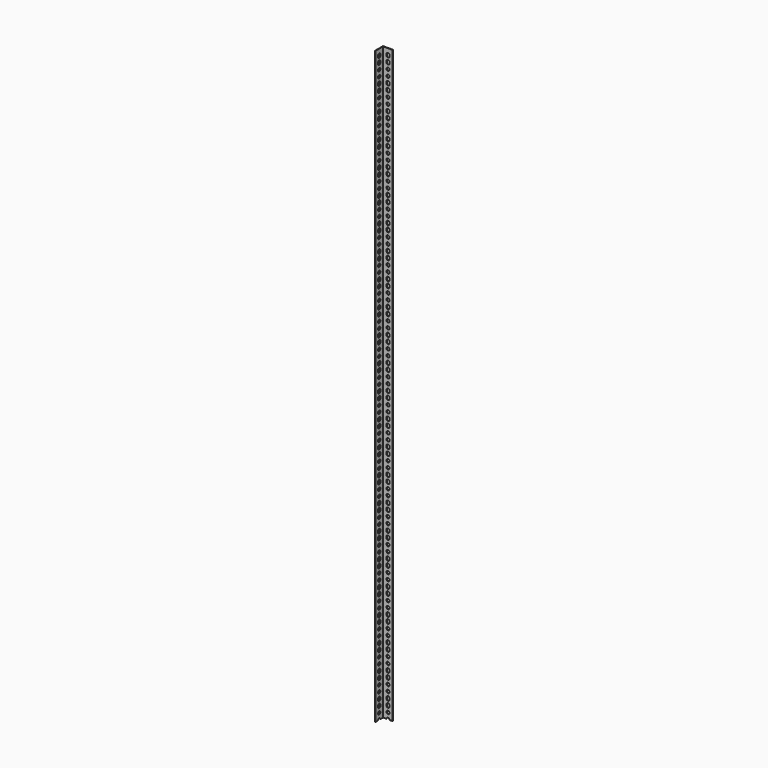
from build123d import *

# Parameters (mm, degrees)
F2_DEPTH = 1828.8
F3_R     = 4.7625
F5_DEPTH = 1.3726
F4_R     = 4.7625
F6_DEPTH = 1.3726


# Not quite as in the source:
# - a variable given as a bare number and used for a length is read in inches; the dataset says mm whatever the document's units were


with BuildPart() as f2:
    # F1 (on Top) → F2 (new body)
    with BuildSketch(Plane.XY):
        Polygon((-1.3716, 1.3716), (-1.3716, -28.7528), (0, -28.7528), (0, 0), (28.7528, 0), (28.7528, 1.3716), align=None)
    extrude(amount=F2_DEPTH)

    # F3 (on face) → F5 (cut, through all)
    with BuildSketch(Plane.XZ):
        with Locations((15.1384, 19.05)):
            Circle(F3_R)
        with Locations((15.1384, 0)):
            Circle(F3_R)
        with BuildLine():
            Line((19.9009, 36.5125), (19.9009, 39.6875))
            ThreePointArc((19.9009, 39.6875), (15.1384, 44.45), (10.3759, 39.6875))
            Line((10.3759, 39.6875), (10.3759, 36.5125))
            ThreePointArc((10.3759, 36.5125), (15.1384, 31.75), (19.9009, 36.5125))
        make_face()
        with BuildLine():
            Line((19.9009, 55.5625), (19.9009, 58.7375))
            ThreePointArc((19.9009, 58.7375), (15.1384, 63.5), (10.3759, 58.7375))
            Line((10.3759, 58.7375), (10.3759, 55.5625))
            ThreePointArc((10.3759, 55.5625), (15.1384, 50.8), (19.9009, 55.5625))
        make_face()
        with BuildLine():
            Line((19.9009, 131.7625), (19.9009, 134.9375))
            ThreePointArc((19.9009, 134.9375), (15.1384, 139.7), (10.3759, 134.9375))
            Line((10.3759, 134.9375), (10.3759, 131.7625))
            ThreePointArc((10.3759, 131.7625), (15.1384, 127), (19.9009, 131.7625))
        make_face()
        with Locations((15.1384, 95.25)):
            Circle(F3_R)
        with Locations((15.1384, 76.2)):
            Circle(F3_R)
        with BuildLine():
            Line((19.9009, 112.7125), (19.9009, 115.8875))
            ThreePointArc((19.9009, 115.8875), (15.1384, 120.65), (10.3759, 115.8875))
            Line((10.3759, 115.8875), (10.3759, 112.7125))
            ThreePointArc((10.3759, 112.7125), (15.1384, 107.95), (19.9009, 112.7125))
        make_face()
        with BuildLine():
            Line((19.9009, 207.9625), (19.9009, 211.1375))
            ThreePointArc((19.9009, 211.1375), (15.1384, 215.9), (10.3759, 211.1375))
            Line((10.3759, 211.1375), (10.3759, 207.9625))
            ThreePointArc((10.3759, 207.9625), (15.1384, 203.2), (19.9009, 207.9625))
        make_face()
        with Locations((15.1384, 171.45)):
            Circle(F3_R)
        with Locations((15.1384, 152.4)):
            Circle(F3_R)
        with BuildLine():
            Line((19.9009, 188.9125), (19.9009, 192.0875))
            ThreePointArc((19.9009, 192.0875), (15.1384, 196.85), (10.3759, 192.0875))
            Line((10.3759, 192.0875), (10.3759, 188.9125))
            ThreePointArc((10.3759, 188.9125), (15.1384, 184.15), (19.9009, 188.9125))
        make_face()
        with BuildLine():
            Line((19.9009, 284.1625), (19.9009, 287.3375))
            ThreePointArc((19.9009, 287.3375), (15.1384, 292.1), (10.3759, 287.3375))
            Line((10.3759, 287.3375), (10.3759, 284.1625))
            ThreePointArc((10.3759, 284.1625), (15.1384, 279.4), (19.9009, 284.1625))
        make_face()
        with Locations((15.1384, 247.65)):
            Circle(F3_R)
        with Locations((15.1384, 228.6)):
            Circle(F3_R)
        with BuildLine():
            Line((19.9009, 265.1125), (19.9009, 268.2875))
            ThreePointArc((19.9009, 268.2875), (15.1384, 273.05), (10.3759, 268.2875))
            Line((10.3759, 268.2875), (10.3759, 265.1125))
            ThreePointArc((10.3759, 265.1125), (15.1384, 260.35), (19.9009, 265.1125))
        make_face()
        with BuildLine():
            Line((19.9009, 360.3625), (19.9009, 363.5375))
            ThreePointArc((19.9009, 363.5375), (15.1384, 368.3), (10.3759, 363.5375))
            Line((10.3759, 363.5375), (10.3759, 360.3625))
            ThreePointArc((10.3759, 360.3625), (15.1384, 355.6), (19.9009, 360.3625))
        make_face()
        with Locations((15.1384, 323.85)):
            Circle(F3_R)
        with Locations((15.1384, 304.8)):
            Circle(F3_R)
        with BuildLine():
            Line((19.9009, 341.3125), (19.9009, 344.4875))
            ThreePointArc((19.9009, 344.4875), (15.1384, 349.25), (10.3759, 344.4875))
            Line((10.3759, 344.4875), (10.3759, 341.3125))
            ThreePointArc((10.3759, 341.3125), (15.1384, 336.55), (19.9009, 341.3125))
        make_face()
        with BuildLine():
            Line((19.9009, 436.5625), (19.9009, 439.7375))
            ThreePointArc((19.9009, 439.7375), (15.1384, 444.5), (10.3759, 439.7375))
            Line((10.3759, 439.7375), (10.3759, 436.5625))
            ThreePointArc((10.3759, 436.5625), (15.1384, 431.8), (19.9009, 436.5625))
        make_face()
        with Locations((15.1384, 400.05)):
            Circle(F3_R)
        with Locations((15.1384, 381)):
            Circle(F3_R)
        with BuildLine():
            Line((19.9009, 417.5125), (19.9009, 420.6875))
            ThreePointArc((19.9009, 420.6875), (15.1384, 425.45), (10.3759, 420.6875))
            Line((10.3759, 420.6875), (10.3759, 417.5125))
            ThreePointArc((10.3759, 417.5125), (15.1384, 412.75), (19.9009, 417.5125))
        make_face()
        with BuildLine():
            Line((19.9009, 512.7625), (19.9009, 515.9375))
            ThreePointArc((19.9009, 515.9375), (15.1384, 520.7), (10.3759, 515.9375))
            Line((10.3759, 515.9375), (10.3759, 512.7625))
            ThreePointArc((10.3759, 512.7625), (15.1384, 508), (19.9009, 512.7625))
        make_face()
        with Locations((15.1384, 476.25)):
            Circle(F3_R)
        with Locations((15.1384, 457.2)):
            Circle(F3_R)
        with BuildLine():
            Line((19.9009, 493.7125), (19.9009, 496.8875))
            ThreePointArc((19.9009, 496.8875), (15.1384, 501.65), (10.3759, 496.8875))
            Line((10.3759, 496.8875), (10.3759, 493.7125))
            ThreePointArc((10.3759, 493.7125), (15.1384, 488.95), (19.9009, 493.7125))
        make_face()
        with BuildLine():
            Line((19.9009, 588.9625), (19.9009, 592.1375))
            ThreePointArc((19.9009, 592.1375), (15.1384, 596.9), (10.3759, 592.1375))
            Line((10.3759, 592.1375), (10.3759, 588.9625))
            ThreePointArc((10.3759, 588.9625), (15.1384, 584.2), (19.9009, 588.9625))
        make_face()
        with Locations((15.1384, 552.45)):
            Circle(F3_R)
        with Locations((15.1384, 533.4)):
            Circle(F3_R)
        with BuildLine():
            Line((19.9009, 569.9125), (19.9009, 573.0875))
            ThreePointArc((19.9009, 573.0875), (15.1384, 577.85), (10.3759, 573.0875))
            Line((10.3759, 573.0875), (10.3759, 569.9125))
            ThreePointArc((10.3759, 569.9125), (15.1384, 565.15), (19.9009, 569.9125))
        make_face()
        with BuildLine():
            Line((19.9009, 665.1625), (19.9009, 668.3375))
            ThreePointArc((19.9009, 668.3375), (15.1384, 673.1), (10.3759, 668.3375))
            Line((10.3759, 668.3375), (10.3759, 665.1625))
            ThreePointArc((10.3759, 665.1625), (15.1384, 660.4), (19.9009, 665.1625))
        make_face()
        with Locations((15.1384, 628.65)):
            Circle(F3_R)
        with Locations((15.1384, 609.6)):
            Circle(F3_R)
        with BuildLine():
            Line((19.9009, 646.1125), (19.9009, 649.2875))
            ThreePointArc((19.9009, 649.2875), (15.1384, 654.05), (10.3759, 649.2875))
            Line((10.3759, 649.2875), (10.3759, 646.1125))
            ThreePointArc((10.3759, 646.1125), (15.1384, 641.35), (19.9009, 646.1125))
        make_face()
        with BuildLine():
            Line((19.9009, 741.3625), (19.9009, 744.5375))
            ThreePointArc((19.9009, 744.5375), (15.1384, 749.3), (10.3759, 744.5375))
            Line((10.3759, 744.5375), (10.3759, 741.3625))
            ThreePointArc((10.3759, 741.3625), (15.1384, 736.6), (19.9009, 741.3625))
        make_face()
        with Locations((15.1384, 704.85)):
            Circle(F3_R)
        with Locations((15.1384, 685.8)):
            Circle(F3_R)
        with BuildLine():
            Line((19.9009, 722.3125), (19.9009, 725.4875))
            ThreePointArc((19.9009, 725.4875), (15.1384, 730.25), (10.3759, 725.4875))
            Line((10.3759, 725.4875), (10.3759, 722.3125))
            ThreePointArc((10.3759, 722.3125), (15.1384, 717.55), (19.9009, 722.3125))
        make_face()
        with BuildLine():
            Line((19.9009, 817.5625), (19.9009, 820.7375))
            ThreePointArc((19.9009, 820.7375), (15.1384, 825.5), (10.3759, 820.7375))
            Line((10.3759, 820.7375), (10.3759, 817.5625))
            ThreePointArc((10.3759, 817.5625), (15.1384, 812.8), (19.9009, 817.5625))
        make_face()
        with Locations((15.1384, 781.05)):
            Circle(F3_R)
        with Locations((15.1384, 762)):
            Circle(F3_R)
        with BuildLine():
            Line((19.9009, 798.5125), (19.9009, 801.6875))
            ThreePointArc((19.9009, 801.6875), (15.1384, 806.45), (10.3759, 801.6875))
            Line((10.3759, 801.6875), (10.3759, 798.5125))
            ThreePointArc((10.3759, 798.5125), (15.1384, 793.75), (19.9009, 798.5125))
        make_face()
        with BuildLine():
            Line((19.9009, 893.7625), (19.9009, 896.9375))
            ThreePointArc((19.9009, 896.9375), (15.1384, 901.7), (10.3759, 896.9375))
            Line((10.3759, 896.9375), (10.3759, 893.7625))
            ThreePointArc((10.3759, 893.7625), (15.1384, 889), (19.9009, 893.7625))
        make_face()
        with Locations((15.1384, 857.25)):
            Circle(F3_R)
        with Locations((15.1384, 838.2)):
            Circle(F3_R)
        with BuildLine():
            Line((19.9009, 874.7125), (19.9009, 877.8875))
            ThreePointArc((19.9009, 877.8875), (15.1384, 882.65), (10.3759, 877.8875))
            Line((10.3759, 877.8875), (10.3759, 874.7125))
            ThreePointArc((10.3759, 874.7125), (15.1384, 869.95), (19.9009, 874.7125))
        make_face()
        with BuildLine():
            Line((19.9009, 969.9625), (19.9009, 973.1375))
            ThreePointArc((19.9009, 973.1375), (15.1384, 977.9), (10.3759, 973.1375))
            Line((10.3759, 973.1375), (10.3759, 969.9625))
            ThreePointArc((10.3759, 969.9625), (15.1384, 965.2), (19.9009, 969.9625))
        make_face()
        with Locations((15.1384, 933.45)):
            Circle(F3_R)
        with Locations((15.1384, 914.4)):
            Circle(F3_R)
        with BuildLine():
            Line((19.9009, 950.9125), (19.9009, 954.0875))
            ThreePointArc((19.9009, 954.0875), (15.1384, 958.85), (10.3759, 954.0875))
            Line((10.3759, 954.0875), (10.3759, 950.9125))
            ThreePointArc((10.3759, 950.9125), (15.1384, 946.15), (19.9009, 950.9125))
        make_face()
        with BuildLine():
            Line((19.9009, 1046.1625), (19.9009, 1049.3375))
            ThreePointArc((19.9009, 1049.3375), (15.1384, 1054.1), (10.3759, 1049.3375))
            Line((10.3759, 1049.3375), (10.3759, 1046.1625))
            ThreePointArc((10.3759, 1046.1625), (15.1384, 1041.4), (19.9009, 1046.1625))
        make_face()
        with Locations((15.1384, 1009.65)):
            Circle(F3_R)
        with Locations((15.1384, 990.6)):
            Circle(F3_R)
        with BuildLine():
            Line((19.9009, 1027.1125), (19.9009, 1030.2875))
            ThreePointArc((19.9009, 1030.2875), (15.1384, 1035.05), (10.3759, 1030.2875))
            Line((10.3759, 1030.2875), (10.3759, 1027.1125))
            ThreePointArc((10.3759, 1027.1125), (15.1384, 1022.35), (19.9009, 1027.1125))
        make_face()
        with BuildLine():
            Line((19.9009, 1122.3625), (19.9009, 1125.5375))
            ThreePointArc((19.9009, 1125.5375), (15.1384, 1130.3), (10.3759, 1125.5375))
            Line((10.3759, 1125.5375), (10.3759, 1122.3625))
            ThreePointArc((10.3759, 1122.3625), (15.1384, 1117.6), (19.9009, 1122.3625))
        make_face()
        with Locations((15.1384, 1085.85)):
            Circle(F3_R)
        with Locations((15.1384, 1066.8)):
            Circle(F3_R)
        with BuildLine():
            Line((19.9009, 1103.3125), (19.9009, 1106.4875))
            ThreePointArc((19.9009, 1106.4875), (15.1384, 1111.25), (10.3759, 1106.4875))
            Line((10.3759, 1106.4875), (10.3759, 1103.3125))
            ThreePointArc((10.3759, 1103.3125), (15.1384, 1098.55), (19.9009, 1103.3125))
        make_face()
        with BuildLine():
            Line((19.9009, 1198.5625), (19.9009, 1201.7375))
            ThreePointArc((19.9009, 1201.7375), (15.1384, 1206.5), (10.3759, 1201.7375))
            Line((10.3759, 1201.7375), (10.3759, 1198.5625))
            ThreePointArc((10.3759, 1198.5625), (15.1384, 1193.8), (19.9009, 1198.5625))
        make_face()
        with Locations((15.1384, 1162.05)):
            Circle(F3_R)
        with Locations((15.1384, 1143)):
            Circle(F3_R)
        with BuildLine():
            Line((19.9009, 1179.5125), (19.9009, 1182.6875))
            ThreePointArc((19.9009, 1182.6875), (15.1384, 1187.45), (10.3759, 1182.6875))
            Line((10.3759, 1182.6875), (10.3759, 1179.5125))
            ThreePointArc((10.3759, 1179.5125), (15.1384, 1174.75), (19.9009, 1179.5125))
        make_face()
        with BuildLine():
            Line((19.9009, 1274.7625), (19.9009, 1277.9375))
            ThreePointArc((19.9009, 1277.9375), (15.1384, 1282.7), (10.3759, 1277.9375))
            Line((10.3759, 1277.9375), (10.3759, 1274.7625))
            ThreePointArc((10.3759, 1274.7625), (15.1384, 1270), (19.9009, 1274.7625))
        make_face()
        with Locations((15.1384, 1238.25)):
            Circle(F3_R)
        with Locations((15.1384, 1219.2)):
            Circle(F3_R)
        with BuildLine():
            Line((19.9009, 1255.7125), (19.9009, 1258.8875))
            ThreePointArc((19.9009, 1258.8875), (15.1384, 1263.65), (10.3759, 1258.8875))
            Line((10.3759, 1258.8875), (10.3759, 1255.7125))
            ThreePointArc((10.3759, 1255.7125), (15.1384, 1250.95), (19.9009, 1255.7125))
        make_face()
        with BuildLine():
            Line((19.9009, 1350.9625), (19.9009, 1354.1375))
            ThreePointArc((19.9009, 1354.1375), (15.1384, 1358.9), (10.3759, 1354.1375))
            Line((10.3759, 1354.1375), (10.3759, 1350.9625))
            ThreePointArc((10.3759, 1350.9625), (15.1384, 1346.2), (19.9009, 1350.9625))
        make_face()
        with Locations((15.1384, 1314.45)):
            Circle(F3_R)
        with Locations((15.1384, 1295.4)):
            Circle(F3_R)
        with BuildLine():
            Line((19.9009, 1331.9125), (19.9009, 1335.0875))
            ThreePointArc((19.9009, 1335.0875), (15.1384, 1339.85), (10.3759, 1335.0875))
            Line((10.3759, 1335.0875), (10.3759, 1331.9125))
            ThreePointArc((10.3759, 1331.9125), (15.1384, 1327.15), (19.9009, 1331.9125))
        make_face()
        with BuildLine():
            Line((19.9009, 1427.1625), (19.9009, 1430.3375))
            ThreePointArc((19.9009, 1430.3375), (15.1384, 1435.1), (10.3759, 1430.3375))
            Line((10.3759, 1430.3375), (10.3759, 1427.1625))
            ThreePointArc((10.3759, 1427.1625), (15.1384, 1422.4), (19.9009, 1427.1625))
        make_face()
        with Locations((15.1384, 1390.65)):
            Circle(F3_R)
        with Locations((15.1384, 1371.6)):
            Circle(F3_R)
        with BuildLine():
            Line((19.9009, 1408.1125), (19.9009, 1411.2875))
            ThreePointArc((19.9009, 1411.2875), (15.1384, 1416.05), (10.3759, 1411.2875))
            Line((10.3759, 1411.2875), (10.3759, 1408.1125))
            ThreePointArc((10.3759, 1408.1125), (15.1384, 1403.35), (19.9009, 1408.1125))
        make_face()
        with BuildLine():
            Line((19.9009, 1503.3625), (19.9009, 1506.5375))
            ThreePointArc((19.9009, 1506.5375), (15.1384, 1511.3), (10.3759, 1506.5375))
            Line((10.3759, 1506.5375), (10.3759, 1503.3625))
            ThreePointArc((10.3759, 1503.3625), (15.1384, 1498.6), (19.9009, 1503.3625))
        make_face()
        with Locations((15.1384, 1466.85)):
            Circle(F3_R)
        with Locations((15.1384, 1447.8)):
            Circle(F3_R)
        with BuildLine():
            Line((19.9009, 1484.3125), (19.9009, 1487.4875))
            ThreePointArc((19.9009, 1487.4875), (15.1384, 1492.25), (10.3759, 1487.4875))
            Line((10.3759, 1487.4875), (10.3759, 1484.3125))
            ThreePointArc((10.3759, 1484.3125), (15.1384, 1479.55), (19.9009, 1484.3125))
        make_face()
        with BuildLine():
            Line((19.9009, 1579.5625), (19.9009, 1582.7375))
            ThreePointArc((19.9009, 1582.7375), (15.1384, 1587.5), (10.3759, 1582.7375))
            Line((10.3759, 1582.7375), (10.3759, 1579.5625))
            ThreePointArc((10.3759, 1579.5625), (15.1384, 1574.8), (19.9009, 1579.5625))
        make_face()
        with Locations((15.1384, 1543.05)):
            Circle(F3_R)
        with Locations((15.1384, 1524)):
            Circle(F3_R)
        with BuildLine():
            Line((19.9009, 1560.5125), (19.9009, 1563.6875))
            ThreePointArc((19.9009, 1563.6875), (15.1384, 1568.45), (10.3759, 1563.6875))
            Line((10.3759, 1563.6875), (10.3759, 1560.5125))
            ThreePointArc((10.3759, 1560.5125), (15.1384, 1555.75), (19.9009, 1560.5125))
        make_face()
        with BuildLine():
            Line((19.9009, 1655.7625), (19.9009, 1658.9375))
            ThreePointArc((19.9009, 1658.9375), (15.1384, 1663.7), (10.3759, 1658.9375))
            Line((10.3759, 1658.9375), (10.3759, 1655.7625))
            ThreePointArc((10.3759, 1655.7625), (15.1384, 1651), (19.9009, 1655.7625))
        make_face()
        with Locations((15.1384, 1619.25)):
            Circle(F3_R)
        with Locations((15.1384, 1600.2)):
            Circle(F3_R)
        with BuildLine():
            Line((19.9009, 1636.7125), (19.9009, 1639.8875))
            ThreePointArc((19.9009, 1639.8875), (15.1384, 1644.65), (10.3759, 1639.8875))
            Line((10.3759, 1639.8875), (10.3759, 1636.7125))
            ThreePointArc((10.3759, 1636.7125), (15.1384, 1631.95), (19.9009, 1636.7125))
        make_face()
        with BuildLine():
            Line((19.9009, 1731.9625), (19.9009, 1735.1375))
            ThreePointArc((19.9009, 1735.1375), (15.1384, 1739.9), (10.3759, 1735.1375))
            Line((10.3759, 1735.1375), (10.3759, 1731.9625))
            ThreePointArc((10.3759, 1731.9625), (15.1384, 1727.2), (19.9009, 1731.9625))
        make_face()
        with Locations((15.1384, 1695.45)):
            Circle(F3_R)
        with Locations((15.1384, 1676.4)):
            Circle(F3_R)
        with BuildLine():
            Line((19.9009, 1712.9125), (19.9009, 1716.0875))
            ThreePointArc((19.9009, 1716.0875), (15.1384, 1720.85), (10.3759, 1716.0875))
            Line((10.3759, 1716.0875), (10.3759, 1712.9125))
            ThreePointArc((10.3759, 1712.9125), (15.1384, 1708.15), (19.9009, 1712.9125))
        make_face()
        with BuildLine():
            Line((19.9009, 1808.1625), (19.9009, 1811.3375))
            ThreePointArc((19.9009, 1811.3375), (15.1384, 1816.1), (10.3759, 1811.3375))
            Line((10.3759, 1811.3375), (10.3759, 1808.1625))
            ThreePointArc((10.3759, 1808.1625), (15.1384, 1803.4), (19.9009, 1808.1625))
        make_face()
        with Locations((15.1384, 1771.65)):
            Circle(F3_R)
        with Locations((15.1384, 1752.6)):
            Circle(F3_R)
        with BuildLine():
            Line((19.9009, 1789.1125), (19.9009, 1792.2875))
            ThreePointArc((19.9009, 1792.2875), (15.1384, 1797.05), (10.3759, 1792.2875))
            Line((10.3759, 1792.2875), (10.3759, 1789.1125))
            ThreePointArc((10.3759, 1789.1125), (15.1384, 1784.35), (19.9009, 1789.1125))
        make_face()
    extrude(amount=-F5_DEPTH, mode=Mode.SUBTRACT)

    # F4 (on face) → F6 (cut, through all)
    with BuildSketch(Plane.YZ):
        with Locations((-15.1384, 19.05)):
            Circle(F4_R)
        with Locations((-15.1384, 0)):
            Circle(F4_R)
        with BuildLine():
            Line((-10.3759, 36.5125), (-10.3759, 39.6875))
            ThreePointArc((-10.3759, 39.6875), (-15.1384, 44.45), (-19.9009, 39.6875))
            Line((-19.9009, 39.6875), (-19.9009, 36.5125))
            ThreePointArc((-19.9009, 36.5125), (-15.1384, 31.75), (-10.3759, 36.5125))
        make_face()
        with BuildLine():
            Line((-10.3759, 55.5625), (-10.3759, 58.7375))
            ThreePointArc((-10.3759, 58.7375), (-15.1384, 63.5), (-19.9009, 58.7375))
            Line((-19.9009, 58.7375), (-19.9009, 55.5625))
            ThreePointArc((-19.9009, 55.5625), (-15.1384, 50.8), (-10.3759, 55.5625))
        make_face()
        with BuildLine():
            Line((-10.3759, 131.7625), (-10.3759, 134.9375))
            ThreePointArc((-10.3759, 134.9375), (-15.1384, 139.7), (-19.9009, 134.9375))
            Line((-19.9009, 134.9375), (-19.9009, 131.7625))
            ThreePointArc((-19.9009, 131.7625), (-15.1384, 127), (-10.3759, 131.7625))
        make_face()
        with Locations((-15.1384, 95.25)):
            Circle(F4_R)
        with Locations((-15.1384, 76.2)):
            Circle(F4_R)
        with BuildLine():
            Line((-10.3759, 112.7125), (-10.3759, 115.8875))
            ThreePointArc((-10.3759, 115.8875), (-15.1384, 120.65), (-19.9009, 115.8875))
            Line((-19.9009, 115.8875), (-19.9009, 112.7125))
            ThreePointArc((-19.9009, 112.7125), (-15.1384, 107.95), (-10.3759, 112.7125))
        make_face()
        with BuildLine():
            Line((-10.3759, 207.9625), (-10.3759, 211.1375))
            ThreePointArc((-10.3759, 211.1375), (-15.1384, 215.9), (-19.9009, 211.1375))
            Line((-19.9009, 211.1375), (-19.9009, 207.9625))
            ThreePointArc((-19.9009, 207.9625), (-15.1384, 203.2), (-10.3759, 207.9625))
        make_face()
        with Locations((-15.1384, 171.45)):
            Circle(F4_R)
        with Locations((-15.1384, 152.4)):
            Circle(F4_R)
        with BuildLine():
            Line((-10.3759, 188.9125), (-10.3759, 192.0875))
            ThreePointArc((-10.3759, 192.0875), (-15.1384, 196.85), (-19.9009, 192.0875))
            Line((-19.9009, 192.0875), (-19.9009, 188.9125))
            ThreePointArc((-19.9009, 188.9125), (-15.1384, 184.15), (-10.3759, 188.9125))
        make_face()
        with BuildLine():
            Line((-10.3759, 284.1625), (-10.3759, 287.3375))
            ThreePointArc((-10.3759, 287.3375), (-15.1384, 292.1), (-19.9009, 287.3375))
            Line((-19.9009, 287.3375), (-19.9009, 284.1625))
            ThreePointArc((-19.9009, 284.1625), (-15.1384, 279.4), (-10.3759, 284.1625))
        make_face()
        with Locations((-15.1384, 247.65)):
            Circle(F4_R)
        with Locations((-15.1384, 228.6)):
            Circle(F4_R)
        with BuildLine():
            Line((-10.3759, 265.1125), (-10.3759, 268.2875))
            ThreePointArc((-10.3759, 268.2875), (-15.1384, 273.05), (-19.9009, 268.2875))
            Line((-19.9009, 268.2875), (-19.9009, 265.1125))
            ThreePointArc((-19.9009, 265.1125), (-15.1384, 260.35), (-10.3759, 265.1125))
        make_face()
        with BuildLine():
            Line((-10.3759, 360.3625), (-10.3759, 363.5375))
            ThreePointArc((-10.3759, 363.5375), (-15.1384, 368.3), (-19.9009, 363.5375))
            Line((-19.9009, 363.5375), (-19.9009, 360.3625))
            ThreePointArc((-19.9009, 360.3625), (-15.1384, 355.6), (-10.3759, 360.3625))
        make_face()
        with Locations((-15.1384, 323.85)):
            Circle(F4_R)
        with Locations((-15.1384, 304.8)):
            Circle(F4_R)
        with BuildLine():
            Line((-10.3759, 341.3125), (-10.3759, 344.4875))
            ThreePointArc((-10.3759, 344.4875), (-15.1384, 349.25), (-19.9009, 344.4875))
            Line((-19.9009, 344.4875), (-19.9009, 341.3125))
            ThreePointArc((-19.9009, 341.3125), (-15.1384, 336.55), (-10.3759, 341.3125))
        make_face()
        with BuildLine():
            Line((-10.3759, 436.5625), (-10.3759, 439.7375))
            ThreePointArc((-10.3759, 439.7375), (-15.1384, 444.5), (-19.9009, 439.7375))
            Line((-19.9009, 439.7375), (-19.9009, 436.5625))
            ThreePointArc((-19.9009, 436.5625), (-15.1384, 431.8), (-10.3759, 436.5625))
        make_face()
        with Locations((-15.1384, 400.05)):
            Circle(F4_R)
        with Locations((-15.1384, 381)):
            Circle(F4_R)
        with BuildLine():
            Line((-10.3759, 417.5125), (-10.3759, 420.6875))
            ThreePointArc((-10.3759, 420.6875), (-15.1384, 425.45), (-19.9009, 420.6875))
            Line((-19.9009, 420.6875), (-19.9009, 417.5125))
            ThreePointArc((-19.9009, 417.5125), (-15.1384, 412.75), (-10.3759, 417.5125))
        make_face()
        with BuildLine():
            Line((-10.3759, 512.7625), (-10.3759, 515.9375))
            ThreePointArc((-10.3759, 515.9375), (-15.1384, 520.7), (-19.9009, 515.9375))
            Line((-19.9009, 515.9375), (-19.9009, 512.7625))
            ThreePointArc((-19.9009, 512.7625), (-15.1384, 508), (-10.3759, 512.7625))
        make_face()
        with Locations((-15.1384, 476.25)):
            Circle(F4_R)
        with Locations((-15.1384, 457.2)):
            Circle(F4_R)
        with BuildLine():
            Line((-10.3759, 493.7125), (-10.3759, 496.8875))
            ThreePointArc((-10.3759, 496.8875), (-15.1384, 501.65), (-19.9009, 496.8875))
            Line((-19.9009, 496.8875), (-19.9009, 493.7125))
            ThreePointArc((-19.9009, 493.7125), (-15.1384, 488.95), (-10.3759, 493.7125))
        make_face()
        with BuildLine():
            Line((-10.3759, 588.9625), (-10.3759, 592.1375))
            ThreePointArc((-10.3759, 592.1375), (-15.1384, 596.9), (-19.9009, 592.1375))
            Line((-19.9009, 592.1375), (-19.9009, 588.9625))
            ThreePointArc((-19.9009, 588.9625), (-15.1384, 584.2), (-10.3759, 588.9625))
        make_face()
        with Locations((-15.1384, 552.45)):
            Circle(F4_R)
        with Locations((-15.1384, 533.4)):
            Circle(F4_R)
        with BuildLine():
            Line((-10.3759, 569.9125), (-10.3759, 573.0875))
            ThreePointArc((-10.3759, 573.0875), (-15.1384, 577.85), (-19.9009, 573.0875))
            Line((-19.9009, 573.0875), (-19.9009, 569.9125))
            ThreePointArc((-19.9009, 569.9125), (-15.1384, 565.15), (-10.3759, 569.9125))
        make_face()
        with BuildLine():
            Line((-10.3759, 665.1625), (-10.3759, 668.3375))
            ThreePointArc((-10.3759, 668.3375), (-15.1384, 673.1), (-19.9009, 668.3375))
            Line((-19.9009, 668.3375), (-19.9009, 665.1625))
            ThreePointArc((-19.9009, 665.1625), (-15.1384, 660.4), (-10.3759, 665.1625))
        make_face()
        with Locations((-15.1384, 628.65)):
            Circle(F4_R)
        with Locations((-15.1384, 609.6)):
            Circle(F4_R)
        with BuildLine():
            Line((-10.3759, 646.1125), (-10.3759, 649.2875))
            ThreePointArc((-10.3759, 649.2875), (-15.1384, 654.05), (-19.9009, 649.2875))
            Line((-19.9009, 649.2875), (-19.9009, 646.1125))
            ThreePointArc((-19.9009, 646.1125), (-15.1384, 641.35), (-10.3759, 646.1125))
        make_face()
        with BuildLine():
            Line((-10.3759, 741.3625), (-10.3759, 744.5375))
            ThreePointArc((-10.3759, 744.5375), (-15.1384, 749.3), (-19.9009, 744.5375))
            Line((-19.9009, 744.5375), (-19.9009, 741.3625))
            ThreePointArc((-19.9009, 741.3625), (-15.1384, 736.6), (-10.3759, 741.3625))
        make_face()
        with Locations((-15.1384, 704.85)):
            Circle(F4_R)
        with Locations((-15.1384, 685.8)):
            Circle(F4_R)
        with BuildLine():
            Line((-10.3759, 722.3125), (-10.3759, 725.4875))
            ThreePointArc((-10.3759, 725.4875), (-15.1384, 730.25), (-19.9009, 725.4875))
            Line((-19.9009, 725.4875), (-19.9009, 722.3125))
            ThreePointArc((-19.9009, 722.3125), (-15.1384, 717.55), (-10.3759, 722.3125))
        make_face()
        with BuildLine():
            Line((-10.3759, 817.5625), (-10.3759, 820.7375))
            ThreePointArc((-10.3759, 820.7375), (-15.1384, 825.5), (-19.9009, 820.7375))
            Line((-19.9009, 820.7375), (-19.9009, 817.5625))
            ThreePointArc((-19.9009, 817.5625), (-15.1384, 812.8), (-10.3759, 817.5625))
        make_face()
        with Locations((-15.1384, 781.05)):
            Circle(F4_R)
        with Locations((-15.1384, 762)):
            Circle(F4_R)
        with BuildLine():
            Line((-10.3759, 798.5125), (-10.3759, 801.6875))
            ThreePointArc((-10.3759, 801.6875), (-15.1384, 806.45), (-19.9009, 801.6875))
            Line((-19.9009, 801.6875), (-19.9009, 798.5125))
            ThreePointArc((-19.9009, 798.5125), (-15.1384, 793.75), (-10.3759, 798.5125))
        make_face()
        with BuildLine():
            Line((-10.3759, 893.7625), (-10.3759, 896.9375))
            ThreePointArc((-10.3759, 896.9375), (-15.1384, 901.7), (-19.9009, 896.9375))
            Line((-19.9009, 896.9375), (-19.9009, 893.7625))
            ThreePointArc((-19.9009, 893.7625), (-15.1384, 889), (-10.3759, 893.7625))
        make_face()
        with Locations((-15.1384, 857.25)):
            Circle(F4_R)
        with Locations((-15.1384, 838.2)):
            Circle(F4_R)
        with BuildLine():
            Line((-10.3759, 874.7125), (-10.3759, 877.8875))
            ThreePointArc((-10.3759, 877.8875), (-15.1384, 882.65), (-19.9009, 877.8875))
            Line((-19.9009, 877.8875), (-19.9009, 874.7125))
            ThreePointArc((-19.9009, 874.7125), (-15.1384, 869.95), (-10.3759, 874.7125))
        make_face()
        with BuildLine():
            Line((-10.3759, 969.9625), (-10.3759, 973.1375))
            ThreePointArc((-10.3759, 973.1375), (-15.1384, 977.9), (-19.9009, 973.1375))
            Line((-19.9009, 973.1375), (-19.9009, 969.9625))
            ThreePointArc((-19.9009, 969.9625), (-15.1384, 965.2), (-10.3759, 969.9625))
        make_face()
        with Locations((-15.1384, 933.45)):
            Circle(F4_R)
        with Locations((-15.1384, 914.4)):
            Circle(F4_R)
        with BuildLine():
            Line((-10.3759, 950.9125), (-10.3759, 954.0875))
            ThreePointArc((-10.3759, 954.0875), (-15.1384, 958.85), (-19.9009, 954.0875))
            Line((-19.9009, 954.0875), (-19.9009, 950.9125))
            ThreePointArc((-19.9009, 950.9125), (-15.1384, 946.15), (-10.3759, 950.9125))
        make_face()
        with BuildLine():
            Line((-10.3759, 1046.1625), (-10.3759, 1049.3375))
            ThreePointArc((-10.3759, 1049.3375), (-15.1384, 1054.1), (-19.9009, 1049.3375))
            Line((-19.9009, 1049.3375), (-19.9009, 1046.1625))
            ThreePointArc((-19.9009, 1046.1625), (-15.1384, 1041.4), (-10.3759, 1046.1625))
        make_face()
        with Locations((-15.1384, 1009.65)):
            Circle(F4_R)
        with Locations((-15.1384, 990.6)):
            Circle(F4_R)
        with BuildLine():
            Line((-10.3759, 1027.1125), (-10.3759, 1030.2875))
            ThreePointArc((-10.3759, 1030.2875), (-15.1384, 1035.05), (-19.9009, 1030.2875))
            Line((-19.9009, 1030.2875), (-19.9009, 1027.1125))
            ThreePointArc((-19.9009, 1027.1125), (-15.1384, 1022.35), (-10.3759, 1027.1125))
        make_face()
        with BuildLine():
            Line((-10.3759, 1122.3625), (-10.3759, 1125.5375))
            ThreePointArc((-10.3759, 1125.5375), (-15.1384, 1130.3), (-19.9009, 1125.5375))
            Line((-19.9009, 1125.5375), (-19.9009, 1122.3625))
            ThreePointArc((-19.9009, 1122.3625), (-15.1384, 1117.6), (-10.3759, 1122.3625))
        make_face()
        with Locations((-15.1384, 1085.85)):
            Circle(F4_R)
        with Locations((-15.1384, 1066.8)):
            Circle(F4_R)
        with BuildLine():
            Line((-10.3759, 1103.3125), (-10.3759, 1106.4875))
            ThreePointArc((-10.3759, 1106.4875), (-15.1384, 1111.25), (-19.9009, 1106.4875))
            Line((-19.9009, 1106.4875), (-19.9009, 1103.3125))
            ThreePointArc((-19.9009, 1103.3125), (-15.1384, 1098.55), (-10.3759, 1103.3125))
        make_face()
        with BuildLine():
            Line((-10.3759, 1198.5625), (-10.3759, 1201.7375))
            ThreePointArc((-10.3759, 1201.7375), (-15.1384, 1206.5), (-19.9009, 1201.7375))
            Line((-19.9009, 1201.7375), (-19.9009, 1198.5625))
            ThreePointArc((-19.9009, 1198.5625), (-15.1384, 1193.8), (-10.3759, 1198.5625))
        make_face()
        with Locations((-15.1384, 1162.05)):
            Circle(F4_R)
        with Locations((-15.1384, 1143)):
            Circle(F4_R)
        with BuildLine():
            Line((-10.3759, 1179.5125), (-10.3759, 1182.6875))
            ThreePointArc((-10.3759, 1182.6875), (-15.1384, 1187.45), (-19.9009, 1182.6875))
            Line((-19.9009, 1182.6875), (-19.9009, 1179.5125))
            ThreePointArc((-19.9009, 1179.5125), (-15.1384, 1174.75), (-10.3759, 1179.5125))
        make_face()
        with BuildLine():
            Line((-10.3759, 1274.7625), (-10.3759, 1277.9375))
            ThreePointArc((-10.3759, 1277.9375), (-15.1384, 1282.7), (-19.9009, 1277.9375))
            Line((-19.9009, 1277.9375), (-19.9009, 1274.7625))
            ThreePointArc((-19.9009, 1274.7625), (-15.1384, 1270), (-10.3759, 1274.7625))
        make_face()
        with Locations((-15.1384, 1238.25)):
            Circle(F4_R)
        with Locations((-15.1384, 1219.2)):
            Circle(F4_R)
        with BuildLine():
            Line((-10.3759, 1255.7125), (-10.3759, 1258.8875))
            ThreePointArc((-10.3759, 1258.8875), (-15.1384, 1263.65), (-19.9009, 1258.8875))
            Line((-19.9009, 1258.8875), (-19.9009, 1255.7125))
            ThreePointArc((-19.9009, 1255.7125), (-15.1384, 1250.95), (-10.3759, 1255.7125))
        make_face()
        with BuildLine():
            Line((-10.3759, 1350.9625), (-10.3759, 1354.1375))
            ThreePointArc((-10.3759, 1354.1375), (-15.1384, 1358.9), (-19.9009, 1354.1375))
            Line((-19.9009, 1354.1375), (-19.9009, 1350.9625))
            ThreePointArc((-19.9009, 1350.9625), (-15.1384, 1346.2), (-10.3759, 1350.9625))
        make_face()
        with Locations((-15.1384, 1314.45)):
            Circle(F4_R)
        with Locations((-15.1384, 1295.4)):
            Circle(F4_R)
        with BuildLine():
            Line((-10.3759, 1331.9125), (-10.3759, 1335.0875))
            ThreePointArc((-10.3759, 1335.0875), (-15.1384, 1339.85), (-19.9009, 1335.0875))
            Line((-19.9009, 1335.0875), (-19.9009, 1331.9125))
            ThreePointArc((-19.9009, 1331.9125), (-15.1384, 1327.15), (-10.3759, 1331.9125))
        make_face()
        with BuildLine():
            Line((-10.3759, 1427.1625), (-10.3759, 1430.3375))
            ThreePointArc((-10.3759, 1430.3375), (-15.1384, 1435.1), (-19.9009, 1430.3375))
            Line((-19.9009, 1430.3375), (-19.9009, 1427.1625))
            ThreePointArc((-19.9009, 1427.1625), (-15.1384, 1422.4), (-10.3759, 1427.1625))
        make_face()
        with Locations((-15.1384, 1390.65)):
            Circle(F4_R)
        with Locations((-15.1384, 1371.6)):
            Circle(F4_R)
        with BuildLine():
            Line((-10.3759, 1408.1125), (-10.3759, 1411.2875))
            ThreePointArc((-10.3759, 1411.2875), (-15.1384, 1416.05), (-19.9009, 1411.2875))
            Line((-19.9009, 1411.2875), (-19.9009, 1408.1125))
            ThreePointArc((-19.9009, 1408.1125), (-15.1384, 1403.35), (-10.3759, 1408.1125))
        make_face()
        with BuildLine():
            Line((-10.3759, 1503.3625), (-10.3759, 1506.5375))
            ThreePointArc((-10.3759, 1506.5375), (-15.1384, 1511.3), (-19.9009, 1506.5375))
            Line((-19.9009, 1506.5375), (-19.9009, 1503.3625))
            ThreePointArc((-19.9009, 1503.3625), (-15.1384, 1498.6), (-10.3759, 1503.3625))
        make_face()
        with Locations((-15.1384, 1466.85)):
            Circle(F4_R)
        with Locations((-15.1384, 1447.8)):
            Circle(F4_R)
        with BuildLine():
            Line((-10.3759, 1484.3125), (-10.3759, 1487.4875))
            ThreePointArc((-10.3759, 1487.4875), (-15.1384, 1492.25), (-19.9009, 1487.4875))
            Line((-19.9009, 1487.4875), (-19.9009, 1484.3125))
            ThreePointArc((-19.9009, 1484.3125), (-15.1384, 1479.55), (-10.3759, 1484.3125))
        make_face()
        with BuildLine():
            Line((-10.3759, 1579.5625), (-10.3759, 1582.7375))
            ThreePointArc((-10.3759, 1582.7375), (-15.1384, 1587.5), (-19.9009, 1582.7375))
            Line((-19.9009, 1582.7375), (-19.9009, 1579.5625))
            ThreePointArc((-19.9009, 1579.5625), (-15.1384, 1574.8), (-10.3759, 1579.5625))
        make_face()
        with Locations((-15.1384, 1543.05)):
            Circle(F4_R)
        with Locations((-15.1384, 1524)):
            Circle(F4_R)
        with BuildLine():
            Line((-10.3759, 1560.5125), (-10.3759, 1563.6875))
            ThreePointArc((-10.3759, 1563.6875), (-15.1384, 1568.45), (-19.9009, 1563.6875))
            Line((-19.9009, 1563.6875), (-19.9009, 1560.5125))
            ThreePointArc((-19.9009, 1560.5125), (-15.1384, 1555.75), (-10.3759, 1560.5125))
        make_face()
        with BuildLine():
            Line((-10.3759, 1655.7625), (-10.3759, 1658.9375))
            ThreePointArc((-10.3759, 1658.9375), (-15.1384, 1663.7), (-19.9009, 1658.9375))
            Line((-19.9009, 1658.9375), (-19.9009, 1655.7625))
            ThreePointArc((-19.9009, 1655.7625), (-15.1384, 1651), (-10.3759, 1655.7625))
        make_face()
        with Locations((-15.1384, 1619.25)):
            Circle(F4_R)
        with Locations((-15.1384, 1600.2)):
            Circle(F4_R)
        with BuildLine():
            Line((-10.3759, 1636.7125), (-10.3759, 1639.8875))
            ThreePointArc((-10.3759, 1639.8875), (-15.1384, 1644.65), (-19.9009, 1639.8875))
            Line((-19.9009, 1639.8875), (-19.9009, 1636.7125))
            ThreePointArc((-19.9009, 1636.7125), (-15.1384, 1631.95), (-10.3759, 1636.7125))
        make_face()
        with BuildLine():
            Line((-10.3759, 1731.9625), (-10.3759, 1735.1375))
            ThreePointArc((-10.3759, 1735.1375), (-15.1384, 1739.9), (-19.9009, 1735.1375))
            Line((-19.9009, 1735.1375), (-19.9009, 1731.9625))
            ThreePointArc((-19.9009, 1731.9625), (-15.1384, 1727.2), (-10.3759, 1731.9625))
        make_face()
        with Locations((-15.1384, 1695.45)):
            Circle(F4_R)
        with Locations((-15.1384, 1676.4)):
            Circle(F4_R)
        with BuildLine():
            Line((-10.3759, 1712.9125), (-10.3759, 1716.0875))
            ThreePointArc((-10.3759, 1716.0875), (-15.1384, 1720.85), (-19.9009, 1716.0875))
            Line((-19.9009, 1716.0875), (-19.9009, 1712.9125))
            ThreePointArc((-19.9009, 1712.9125), (-15.1384, 1708.15), (-10.3759, 1712.9125))
        make_face()
        with BuildLine():
            Line((-10.3759, 1808.1625), (-10.3759, 1811.3375))
            ThreePointArc((-10.3759, 1811.3375), (-15.1384, 1816.1), (-19.9009, 1811.3375))
            Line((-19.9009, 1811.3375), (-19.9009, 1808.1625))
            ThreePointArc((-19.9009, 1808.1625), (-15.1384, 1803.4), (-10.3759, 1808.1625))
        make_face()
        with Locations((-15.1384, 1771.65)):
            Circle(F4_R)
        with Locations((-15.1384, 1752.6)):
            Circle(F4_R)
        with BuildLine():
            Line((-10.3759, 1789.1125), (-10.3759, 1792.2875))
            ThreePointArc((-10.3759, 1792.2875), (-15.1384, 1797.05), (-19.9009, 1792.2875))
            Line((-19.9009, 1792.2875), (-19.9009, 1789.1125))
            ThreePointArc((-19.9009, 1789.1125), (-15.1384, 1784.35), (-10.3759, 1789.1125))
        make_face()
    extrude(amount=-F6_DEPTH, mode=Mode.SUBTRACT)


solid = f2.part
